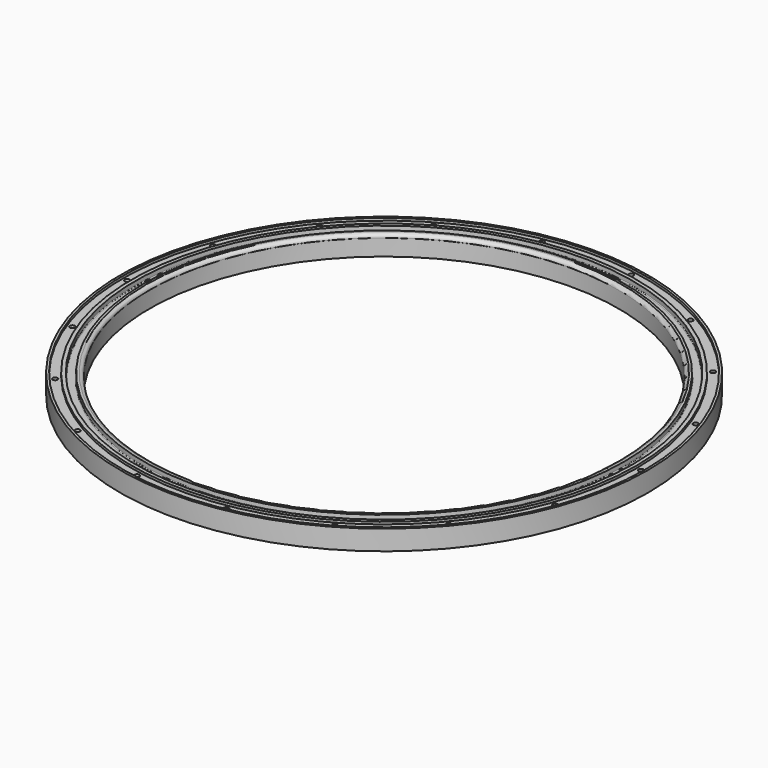
from build123d import *

# Parameters (mm, degrees)
F0_R     = 225
F0_R_2   = 200
F1_DEPTH = 17
F2_R     = 211.9
F2_R_2   = 205
F3_DEPTH = 4
F4_R     = 0.6
F5_R     = 223
F5_R_2   = 215
F6_DEPTH = 2
F7_R     = 3
F9_D     = 4.2
F9_DEPTH = 8.6
F9_TIP   = 1.2618073


# Not quite as in the source:
# - a feature names something its author has since deleted; it is built from what else it names


with BuildPart() as f1:
    # F0 (on Top) → F1 (new body)
    with BuildSketch(Plane.XY):
        Circle(F0_R)
        Circle(F0_R_2, mode=Mode.SUBTRACT)
    extrude(amount=F1_DEPTH)

    # F2 (on face) → F3 (cut)
    with BuildSketch(Plane.XY.offset(17)):
        Circle(F2_R)
        Circle(F2_R_2, mode=Mode.SUBTRACT)
    extrude(amount=-F3_DEPTH, mode=Mode.SUBTRACT)

    # F4
    f4_edges = [f1.edges().sort_by_distance(p)[0] for p in [
        (-211.9, 0, 13),
        (-205, 0, 13),
    ]]
    fillet(f4_edges, radius=F4_R)

    # F5 (on face) → F6 (cut)
    with BuildSketch(Plane.XY.offset(17)):
        Circle(F5_R)
        Circle(F5_R_2, mode=Mode.SUBTRACT)
    extrude(amount=-F6_DEPTH, mode=Mode.SUBTRACT)

    # F7
    f7_edges = [f1.edges().sort_by_distance(p)[0] for p in [
        (-200, 0, 17),
    ]]
    fillet(f7_edges, radius=F7_R)

    # F9
    with Locations(Plane.XY.offset(15)):
        with Locations((219, 0), (205.7926839521, 74.9024113883), (167.7637330431, 140.7704865214), (109.5, 189.6595634288), (38.0289509091, 215.6728979097), (-38.0289509091, 215.6728979097), (-109.5, 189.6595634288), (-167.7637330431, 140.7704865214), (-205.7926839521, 74.9024113883), (-219, 0), (-205.7926839521, -74.9024113883), (-167.7637330431, -140.7704865214), (-109.5, -189.6595634288), (-38.0289509091, -215.6728979097), (38.0289509091, -215.6728979097), (109.5, -189.6595634288), (167.7637330431, -140.7704865214), (205.7926839521, -74.9024113883)):
            Hole(F9_D / 2, depth=F9_DEPTH)
            with Locations((0, 0, -(F9_DEPTH + F9_TIP / 2))):  # 118° drill point
                Cone(0, F9_D / 2, F9_TIP, mode=Mode.SUBTRACT)


solid = f1.part
